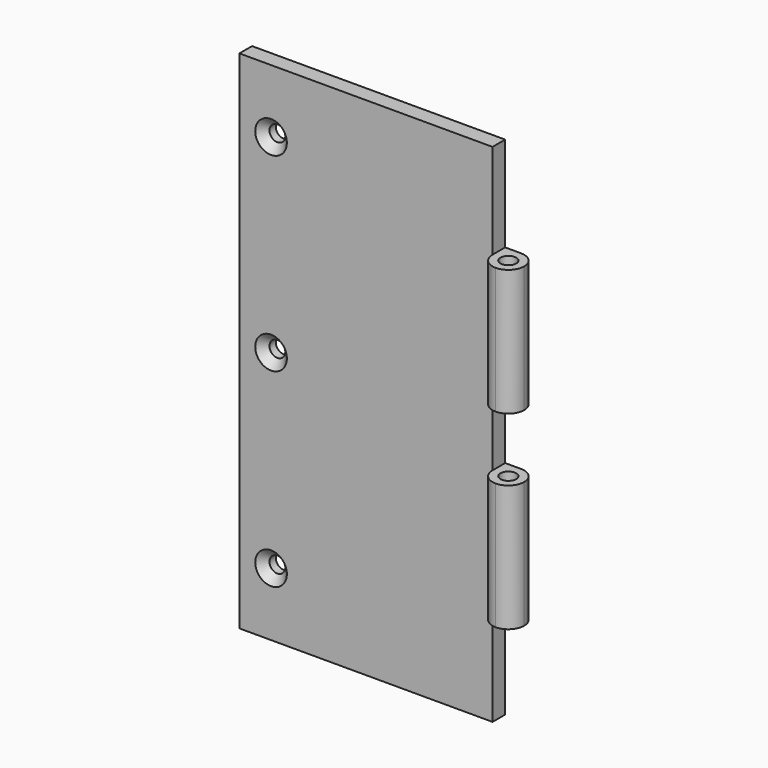
from build123d import *

# Parameters (mm, degrees)
F0_W           = 50.8
F0_H           = 101.6
F1_DEPTH       = 3.175
F2_W           = 6.35
F2_H           = 25.4
F3_DEPTH       = 6.35
F5_DEPTH       = 82.551
F6_R           = 1.5875
F7_DEPTH       = 82.551
F9_D           = 3.175
F9_CSINK_D     = 6.35
F9_CSINK_ANGLE = 90


with BuildPart() as f1:
    # F0 (on Front) → F1 (new body)
    with BuildSketch(Plane.XZ):
        Rectangle(F0_W, F0_H)
    extrude(amount=F1_DEPTH)

    # F2 (on face) → F3 (join)
    with BuildSketch(Plane.YZ.offset(25.4)):
        with Locations((-3.175, 19.05)):
            Rectangle(F2_W, F2_H)
        with Locations((-3.175, -19.05)):
            Rectangle(F2_W, F2_H)
    extrude(amount=F3_DEPTH)

    # F4 (on face) → F5 (cut, through all)
    with BuildSketch(Plane.XY.offset(31.75)):
        with BuildLine():
            Line((31.75, -6.35), (31.75, -3.175))
            ThreePointArc((31.75, -3.175), (30.8200640303, -5.4200640303), (28.575, -6.35))
            Line((28.575, -6.35), (31.75, -6.35))
        make_face()
        with BuildLine():
            ThreePointArc((28.575, 0), (30.8200640303, -0.9299359697), (31.75, -3.175))
            Line((31.75, -3.175), (31.75, 0))
            Line((31.75, 0), (28.575, 0))
        make_face()
        with BuildLine():
            Line((25.4, -6.35), (28.575, -6.35))
            ThreePointArc((28.575, -6.35), (26.3299359697, -5.4200640303), (25.4, -3.175))
            Line((25.4, -3.175), (25.4, -6.35))
        make_face()
    extrude(amount=-F5_DEPTH, mode=Mode.SUBTRACT)

    # F6 (on face) → F7 (cut, through all)
    with BuildSketch(Plane.XY.offset(31.75)):
        with Locations((28.575, -3.175)):
            Circle(F6_R)
    extrude(amount=-F7_DEPTH, mode=Mode.SUBTRACT)

    # F9 (through all)
    with Locations(Plane.XZ.offset(3.175)):
        with Locations((-19.05, 38.1), (-19.05, 0), (-19.05, -38.1)):
            CounterSinkHole(F9_D / 2, F9_CSINK_D / 2, counter_sink_angle=F9_CSINK_ANGLE)


solid = f1.part
